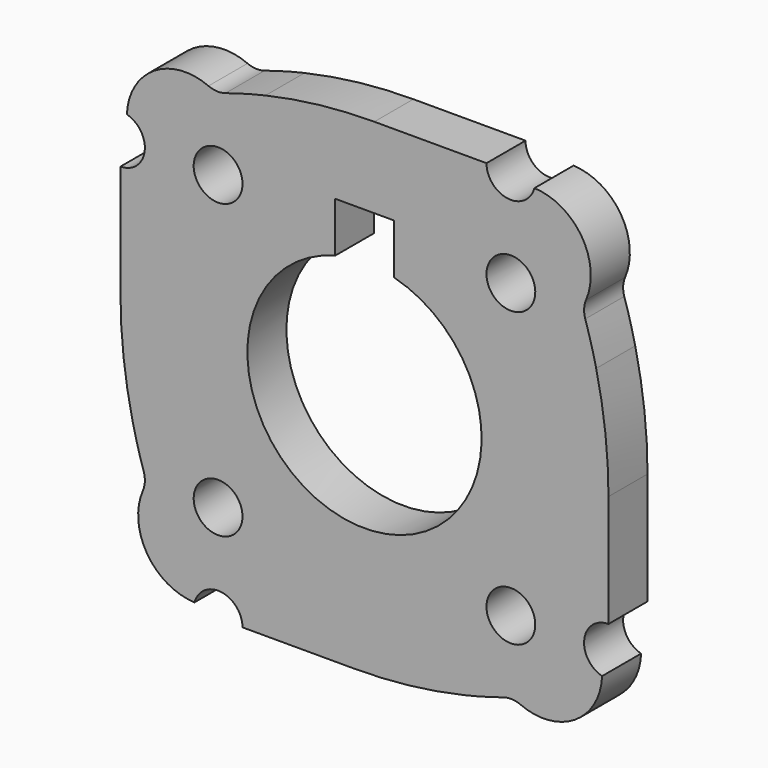
from build123d import *

# Parameters (mm, degrees)
F0_W            = 50
F0_H            = 50
F1_DEPTH        = 5
F2_R            = 2.5
F3_DEPTH        = 25
F3_COPIES_COUNT = 4


# Not quite as in the source:
# - a pattern or mirror of a feature is missing from the dataset's text; its kind, count and spacing are read off the source's solid


with BuildPart() as f1:
    # F0 (on Front) → F1 (new body)
    with BuildSketch(Plane.XZ):
        Rectangle(F0_W, F0_H)
        with BuildLine():
            ThreePointArc((3, 11.6189500386), (0, -12), (-3, 11.6189500386))
            Line((-3, 11.6189500386), (-3, 16.75))
            Line((-3, 16.75), (3, 16.75))
            Line((3, 16.75), (3, 11.6189500386))
        make_face(mode=Mode.SUBTRACT)
    extrude(amount=F1_DEPTH)

    # F2 (on face) → F3 (cut)
    with BuildSketch(Plane.XZ.offset(5)):
        with Locations((-15, 15)):
            Circle(F2_R)
        with BuildLine():
            Line((-25, 25), (-25, 12.5))
            ThreePointArc((-25, 12.5), (-22.5219538073, 14.6694140553), (-24.3446342067, 17.4125703465))
            ThreePointArc((-24.3446342067, 17.4125703465), (-21.5570801866, 22.2577371252), (-15.984957965, 22.7022058824))
            ThreePointArc((-15.984957965, 22.7022058824), (-15.1188510042, 22.5028267103), (-14.2377233051, 22.619047619))
            ThreePointArc((-14.2377233051, 22.619047619), (-12.2019453513, 23.2234626284), (-10.1423385334, 23.7408881171))
            ThreePointArc((-10.1423385334, 23.7408881171), (-4.6026971439, 24.6842248901), (1.0078105936, 25))
            Line((1.0078105936, 25), (-25, 25))
        make_face()
    f3 = extrude(amount=-F3_DEPTH, mode=Mode.SUBTRACT)

    # F3_copies: F3 ×4 about axis
    f3_copies_axis = Axis((0, 0, 0), (0, 1, 0))
    for i in range(1, F3_COPIES_COUNT):
        add(f3.rotate(f3_copies_axis, i * 360 / F3_COPIES_COUNT), mode=Mode.SUBTRACT)


solid = f1.part
